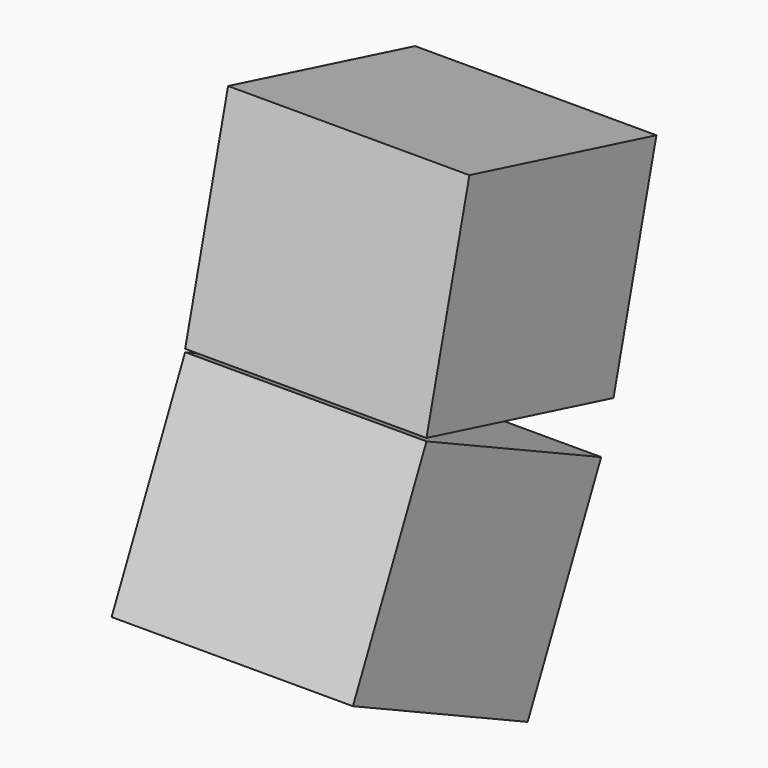
from build123d import *

# Parameters (mm, degrees)
F2_DEPTH = 400


# Not quite as in the source:
# - the program builds the solid bodies; features that only make, move or delete a surface that nothing else refers to are left out


with BuildPart() as f2:
    # F1 (on Right) → F2 (new body, symmetric)
    with BuildSketch(Plane.YZ):
        Polygon((374.981304402, -4201.5043521622), (-400, -4003), (-577.9095256254, -4697.5769940703), (197.0717787767, -4896.0813462325), (286.0265415893, -4548.7928491974), align=None)
    extrude(amount=F2_DEPTH, both=True)


with BuildPart() as f2b:
    # F1 (on Right) → F2, piece 2 (new body, symmetric)
    with BuildSketch(Plane.YZ):
        Polygon((-158.7356341258, -5696.709062444), (-6.28921634, -5372.2366603752), (146.1572014458, -5047.7642583064), (-577.9095256254, -4707.5769940703), (-882.802361197, -5356.5217982079), align=None)
    extrude(amount=F2_DEPTH, both=True)


solid = Compound([f2.part, f2b.part])
